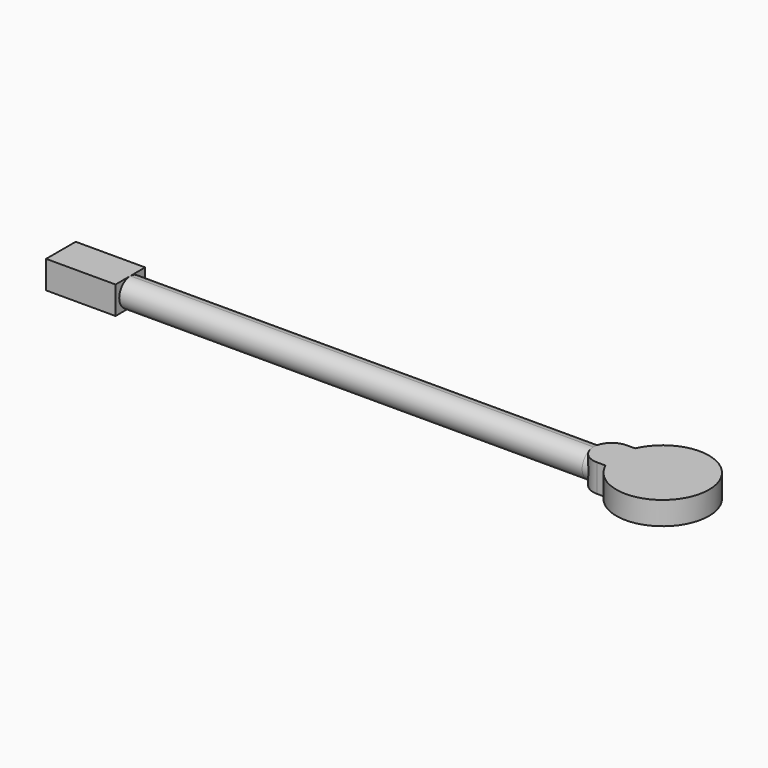
from build123d import *

# Parameters (mm, degrees)
F0_W         = 30
F0_H         = 12
F1_DEPTH     = 16
F3_DEPTH     = 200
F5_DEPTH     = 30
F7_DEPTH     = 10
F8_T4_DEPTH  = 52
F8_S5_R      = 6
F8_T6_DEPTH  = 28
F8_T10_DEPTH = 52
F8_S11_R     = 6
F8_T12_DEPTH = 28
F9_SIZE      = 1.99999


# Not quite as in the source:
# - a fillet or chamfer that OpenCascade refuses, or shapes differently, is made with other operations: its cross-section is extruded or revolved along the edge and cut away or added
# - a fillet or chamfer is up to 0.001 mm smaller than in the source, because OpenCascade refuses the exact size


with BuildPart() as f1:
    # F0 (on Front) → F1 (new body)
    with BuildSketch(Plane.XZ):
        with Locations((15, 6)):
            Rectangle(F0_W, F0_H)
    extrude(amount=F1_DEPTH)

    # F2 (on face) → F3 (join)
    with BuildSketch(Plane.YZ.offset(30)):
        with BuildLine():
            ThreePointArc((-8, 0), (-3.7573593129, 1.7573593129), (-2, 6))
            ThreePointArc((-2, 6), (-3.7573593129, 10.2426406871), (-8, 12))
            ThreePointArc((-8, 12), (-14, 6), (-8, 0))
        make_face()
    extrude(amount=F3_DEPTH)

    # F4 (on face) → F5 (join)
    with BuildSketch(Plane.YZ.offset(230)):
        with BuildLine():
            Line((-8, 12), (-16, 12))
            Line((-16, 12), (-16, 0))
            Line((-16, 0), (-8, 0))
            ThreePointArc((-8, 0), (-14, 6), (-8, 12))
        make_face()
        with BuildLine():
            Line((0, 12), (-8, 12))
            ThreePointArc((-8, 12), (-3.7573593129, 10.2426406871), (-2, 6))
            ThreePointArc((-2, 6), (-3.7573593129, 1.7573593129), (-8, 0))
            Line((-8, 0), (0, 0))
            Line((0, 0), (0, 12))
        make_face()
        with BuildLine():
            ThreePointArc((-2, 6), (-3.7573593129, 10.2426406871), (-8, 12))
            ThreePointArc((-8, 12), (-14, 6), (-8, 0))
            ThreePointArc((-8, 0), (-3.7573593129, 1.7573593129), (-2, 6))
        make_face()
    extrude(amount=F5_DEPTH)

    # F6 (on face) → F7 (join)
    with BuildSketch(Plane.XY.offset(12)):
        with BuildLine():
            ThreePointArc((241.6696972202, -16), (264.0861928738, -27.5781262586), (280, -8))
            ThreePointArc((280, -8), (264.0861928738, 11.5781262586), (241.6696972202, 0))
            Line((241.6696972202, 0), (260, 0))
            Line((260, 0), (260, -16))
            Line((260, -16), (241.6696972202, -16))
        make_face()
    extrude(amount=-F7_DEPTH)

    # F8: fillet of radius 8 on 2 edges, made by hand


with BuildPart() as f8_tool2:
    # F8_s3 → F8_t4 (new body)
    with BuildSketch(Plane.XY.offset(-20)):
        with BuildLine():
            ThreePointArc((230, -8), (232.3431457505, -2.3431457505), (238, 0))
            Line((238, 0), (230, 0))
            Line((230, 0), (230, -8))
        make_face()
    extrude(amount=F8_T4_DEPTH)

    # F8_s5 → F8_t6 (cut, symmetric)
    with BuildSketch(Plane.YZ.offset(234)):
        with Locations((-8, 6)):
            Circle(F8_S5_R)
    extrude(amount=F8_T6_DEPTH, both=True, mode=Mode.SUBTRACT)


with BuildPart() as f1_1:
    add(f1.part)

    # F8_t1: cut F8_tool2
    add(f8_tool2.part, mode=Mode.SUBTRACT)


with BuildPart() as f8_tool8:
    # F8_s9 → F8_t10 (new body)
    with BuildSketch(Plane.XY.offset(32)):
        with BuildLine():
            ThreePointArc((230, -8), (232.3431457505, -13.6568542495), (238, -16))
            Line((238, -16), (230, -16))
            Line((230, -16), (230, -8))
        make_face()
    extrude(amount=-F8_T10_DEPTH)

    # F8_s11 → F8_t12 (cut, symmetric)
    with BuildSketch(Plane.YZ.offset(234)):
        with Locations((-8, 6)):
            Circle(F8_S11_R)
    extrude(amount=F8_T12_DEPTH, both=True, mode=Mode.SUBTRACT)


with BuildPart() as f1_2:
    add(f1_1.part)

    # F8_t7: cut F8_tool8
    add(f8_tool8.part, mode=Mode.SUBTRACT)

    # F9 (size 2 in the source; OpenCascade refuses exactly that, so slightly less here)
    f9_edges = [f1_2.edges().sort_by_distance(p)[0] for p in [
        (260, -8, 0),
    ]]
    chamfer(f9_edges, length=F9_SIZE)


solid = f1_2.part
